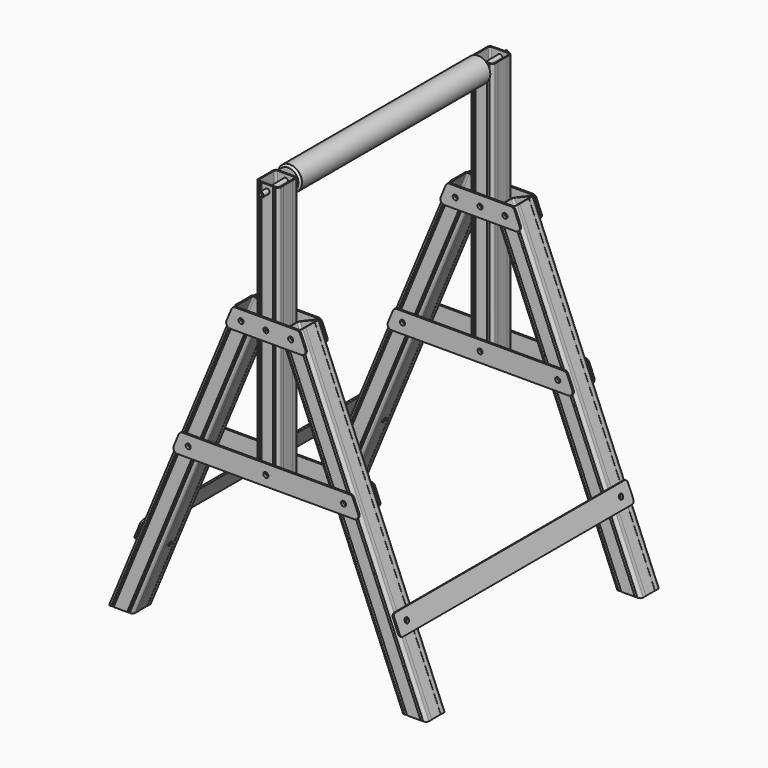
from build123d import *

# Parameters (mm, degrees)
F0_R      = 6.25
F1_DEPTH  = 60
F2_R      = 7.5
F4_REACH  = 887.042655099
F5_R      = 6.25
F6_DEPTH  = 57.7
F7_W      = 55.7
F7_H      = 653.8274706661
F7_R      = 6.25
F8_DEPTH  = 60
F9_R      = 7.5
F11_DEPTH = 653.8274706661
F14_R     = 6.25
F15_DEPTH = 4
F16_R     = 10
F16_2_R   = 10
F21_R     = 5.9
F22_DEPTH = 380
F23_R     = 30
F23_R_2   = 6.25
F24_DEPTH = 295
F25_SIZE  = 2
F26_SIZE  = 5
F28_W     = 720
F28_H     = 50
F28_R     = 6.25
F29_DEPTH = 4
F30_R     = 7.5


# Not quite as in the source:
# - a feature names something its author has since deleted; it is built from what else it names


with BuildPart() as f1:
    # F0 (on Front) → F1 (new body)
    with BuildSketch(Plane.XZ):
        Polygon((-62.4540299569, 0), (0, 0), (-310.7389470805, 750.1901803992), (-364.0467961064, 728.1093463517), align=None)
        with Locations((-201.5402531038, 411.1725293339)):
            Circle(F0_R, mode=Mode.SUBTRACT)
        with Locations((-331.6526201079, 725.2915703878)):
            Circle(F0_R, mode=Mode.SUBTRACT)
    extrude(amount=F1_DEPTH)

    # F2
    f2_edges = [f1.edges().sort_by_distance(p)[0] for p in [
        (-155.369474, -60, 375.09509),
        (-213.250413, -60, 364.054673),
        (-155.369474, 0, 375.09509),
        (-213.250413, 0, 364.054673),
    ]]
    fillet(f2_edges, radius=F2_R)

    f4_end = f1.faces().sort_by_distance((-31.2270149784, -30, 0))[0]
    # F3 (on face) → F4 (cut, up to a face of the model that its end follows)
    with BuildSketch(Plane(origin=(-310.7389470805, 0, 750.1901803992), x_dir=(0.9238795325, 0, 0.3826834324), z_dir=(-0.3826834324, 0, 0.9238795325))):
        with BuildLine():
            Line((-54.8, -30), (-54.8, -52.5))
            ThreePointArc((-54.8, -52.5), (-53.4526911935, -55.7526911935), (-50.2, -57.1))
            Line((-50.2, -57.1), (-28.85, -57.1))
            Line((-28.85, -57.1), (-7.5, -57.1))
            ThreePointArc((-7.5, -57.1), (-4.2473088065, -55.7526911935), (-2.9, -52.5))
            Line((-2.9, -52.5), (-2.9, -30))
            Line((-2.9, -30), (-2.9, -7.5))
            ThreePointArc((-2.9, -7.5), (-4.2473088065, -4.2473088065), (-7.5, -2.9))
            Line((-7.5, -2.9), (-28.85, -2.9))
            Line((-28.85, -2.9), (-50.2, -2.9))
            ThreePointArc((-50.2, -2.9), (-53.4526911935, -4.2473088065), (-54.8, -7.5))
            Line((-54.8, -7.5), (-54.8, -30))
        make_face()
        Polygon((-44.2, 0), (-46.2, 0), (-45.2, -1), align=None)
        Polygon((-46.2, 0), (-48.2, 0), (-47.2, -1), align=None)
        Polygon((-48.2, 0), (-50.2, 0), (-49.2, -1), align=None)
        Polygon((-57.7, -16), (-57.7, -44), (-57.4, -44), (-57.4, -30), (-57.4, -16), align=None)
        Polygon((-49.2, -59), (-50.2, -60), (-48.2, -60), align=None)
        Polygon((-47.2, -59), (-48.2, -60), (-46.2, -60), align=None)
        Polygon((-45.2, -59), (-46.2, -60), (-44.2, -60), align=None)
        Polygon((-8.5, -59), (-9.5, -60), (-7.5, -60), align=None)
        Polygon((-10.5, -59), (-11.5, -60), (-9.5, -60), align=None)
        Polygon((-12.5, -59), (-13.5, -60), (-11.5, -60), align=None)
        Polygon((-0.3, -44), (0, -44), (0, -16), (-0.3, -16), (-0.3, -30), align=None)
        Polygon((-7.5, 0), (-9.5, 0), (-8.5, -1), align=None)
        Polygon((-9.5, 0), (-11.5, 0), (-10.5, -1), align=None)
        Polygon((-11.5, 0), (-13.5, 0), (-12.5, -1), align=None)
    f4_long = extrude(amount=-F4_REACH, mode=Mode.PRIVATE)
    add(split(f4_long, bisect_by=f4_end, keep=Keep.BOTTOM, mode=Mode.PRIVATE), mode=Mode.SUBTRACT)

    # F5 (on face) → F6 (cut, through all)
    with BuildSketch(Plane(origin=(0, 0, 0), x_dir=(0, 1, 0), z_dir=(0.9238795325, 0, 0.3826834324))):
        with Locations((-30, 200)):
            Circle(F5_R)
    extrude(amount=-F6_DEPTH, mode=Mode.SUBTRACT)


with BuildPart() as f8:
    # F7 (on face) → F8 (new body)
    with BuildSketch(Plane.XZ.offset(60)):
        with Locations((-392.8967961064, 713.086264667)):
            Rectangle(F7_W, F7_H)
        with Locations((-392.8967961064, 411.1725293339)):
            Circle(F7_R, mode=Mode.SUBTRACT)
        with Locations((-392.8967961064, 725.2915703878)):
            Circle(F7_R, mode=Mode.SUBTRACT)
        with Locations((-392.8967961064, 1025)):
            Circle(F7_R, mode=Mode.SUBTRACT)
    extrude(amount=-F8_DEPTH)

    # F9
    f9_edges = [f8.edges().sort_by_distance(p)[0] for p in [
        (-420.746796, -60, 713.086265),
        (-365.046796, -60, 713.086265),
        (-365.046796, 0, 713.086265),
        (-420.746796, 0, 713.086265),
    ]]
    fillet(f9_edges, radius=F9_R)

    # F10 (on face) → F11 (cut, through all)
    with BuildSketch(Plane.XY.offset(1040)):
        Polygon((-412.2467961064, -59), (-413.2467961064, -60), (-411.2467961064, -60), align=None)
        Polygon((-410.2467961064, -59), (-411.2467961064, -60), (-409.2467961064, -60), align=None)
        Polygon((-408.2467961064, -59), (-409.2467961064, -60), (-407.2467961064, -60), align=None)
        Polygon((-377.5467961064, -59), (-378.5467961064, -60), (-376.5467961064, -60), align=None)
        Polygon((-375.5467961064, -59), (-376.5467961064, -60), (-374.5467961064, -60), align=None)
        Polygon((-373.5467961064, -59), (-374.5467961064, -60), (-372.5467961064, -60), align=None)
        Polygon((-420.7467961064, -16), (-420.7467961064, -44), (-420.4467961064, -44), (-420.4467961064, -30), (-420.4467961064, -16), align=None)
        Polygon((-365.3467961064, -44), (-365.0467961064, -44), (-365.0467961064, -16), (-365.3467961064, -16), (-365.3467961064, -30), align=None)
        Polygon((-376.5467961064, 0), (-378.5467961064, 0), (-377.5467961064, -1), align=None)
        Polygon((-374.5467961064, 0), (-376.5467961064, 0), (-375.5467961064, -1), align=None)
        Polygon((-372.5467961064, 0), (-374.5467961064, 0), (-373.5467961064, -1), align=None)
        Polygon((-411.2467961064, 0), (-413.2467961064, 0), (-412.2467961064, -1), align=None)
        Polygon((-409.2467961064, 0), (-411.2467961064, 0), (-410.2467961064, -1), align=None)
        Polygon((-407.2467961064, 0), (-409.2467961064, 0), (-408.2467961064, -1), align=None)
        with BuildLine():
            Line((-417.8467961064, -30), (-417.8467961064, -52.5))
            ThreePointArc((-417.8467961064, -52.5), (-416.4994872998, -55.7526911935), (-413.2467961064, -57.1))
            Line((-413.2467961064, -57.1), (-392.8967961064, -57.1))
            Line((-392.8967961064, -57.1), (-372.5467961064, -57.1))
            ThreePointArc((-372.5467961064, -57.1), (-369.2941049129, -55.7526911935), (-367.9467961064, -52.5))
            Line((-367.9467961064, -52.5), (-367.9467961064, -30))
            Line((-367.9467961064, -30), (-367.9467961064, -7.5))
            ThreePointArc((-367.9467961064, -7.5), (-369.2941049129, -4.2473088065), (-372.5467961064, -2.9))
            Line((-372.5467961064, -2.9), (-392.8967961064, -2.9))
            Line((-392.8967961064, -2.9), (-413.2467961064, -2.9))
            ThreePointArc((-413.2467961064, -2.9), (-416.4994872998, -4.2473088065), (-417.8467961064, -7.5))
            Line((-417.8467961064, -7.5), (-417.8467961064, -30))
        make_face()
    extrude(amount=-F11_DEPTH, mode=Mode.SUBTRACT)


with BuildPart() as f13_1:
    # F13: instance of F1
    add(f1.part.mirror(Plane(origin=(-392.8967961064, -30, 713.086264667), x_dir=(0, 1, 0), z_dir=(1, 0, 0))))


with BuildPart() as f15:
    # F14 (on face) → F15 (new body)
    with BuildSketch(Plane.XZ.offset(60)):
        Polygon((-180.6685771847, 436.1725293339), (-605.125015028, 436.1725293339), (-625.8356931467, 386.1725293339), (-159.957899066, 386.1725293339), align=None)
        with Locations((-584.2533391089, 411.1725293339)):
            Circle(F14_R, mode=Mode.SUBTRACT)
        with Locations((-392.8967961064, 411.1725293339)):
            Circle(F14_R, mode=Mode.SUBTRACT)
        with Locations((-201.5402531038, 411.1725293339)):
            Circle(F14_R, mode=Mode.SUBTRACT)
    extrude(amount=F15_DEPTH)

    # F16
    f16_edges = [f15.edges().sort_by_distance(p)[0] for p in [
        (-625.835693, -62, 386.172529),
        (-605.125015, -62, 436.172529),
        (-180.668577, -62, 436.172529),
        (-159.957899, -62, 386.172529),
    ]]
    fillet(f16_edges, radius=F16_R)


with BuildPart() as f15b:
    # F14 (on face) → F15, piece 2 (new body)
    with BuildSketch(Plane.XZ.offset(60)):
        Polygon((-310.7389470805, 750.1901803992), (-475.0546451323, 750.1901803992), (-495.7653232509, 700.1901803992), (-290.0282689618, 700.1901803992), align=None)
        with Locations((-454.1409721048, 725.2915703878)):
            Circle(F14_R, mode=Mode.SUBTRACT)
        with Locations((-392.8967961064, 725.1901803992)):
            Circle(F14_R, mode=Mode.SUBTRACT)
        with Locations((-331.6526201079, 725.2915703878)):
            Circle(F14_R, mode=Mode.SUBTRACT)
    extrude(amount=F15_DEPTH)

    # F16#2
    f16_2_edges = [f15b.edges().sort_by_distance(p)[0] for p in [
        (-475.054645, -62, 750.19018),
        (-495.765323, -62, 700.19018),
        (-310.738947, -62, 750.19018),
        (-290.028269, -62, 700.19018),
    ]]
    fillet(f16_2_edges, radius=F16_2_R)


with BuildPart() as f18_1:
    # F18: instance of F15
    add(f15.part.mirror(Plane(origin=(-392.8967961064, -30, 712.9824259225), x_dir=(1, 0, 0), z_dir=(0, -1, 0))))


with BuildPart() as f18_2:
    # F18: instance of F15b
    add(f15b.part.mirror(Plane(origin=(-392.8967961064, -30, 712.9824259225), x_dir=(1, 0, 0), z_dir=(0, -1, 0))))


with BuildPart() as f20_1:
    # F20: instance of F1
    add(f1.part.mirror(Plane(origin=(-392.8967961064, -360, 712.9381401651), x_dir=(1, 0, 0), z_dir=(0, -1, 0))))


with BuildPart() as f20_2:
    # F20: instance of F18_2
    add(f18_2.part.mirror(Plane(origin=(-392.8967961064, -360, 712.9381401651), x_dir=(1, 0, 0), z_dir=(0, -1, 0))))


with BuildPart() as f20_3:
    # F20: instance of F8
    add(f8.part.mirror(Plane(origin=(-392.8967961064, -360, 712.9381401651), x_dir=(1, 0, 0), z_dir=(0, -1, 0))))


with BuildPart() as f20_4:
    # F20: instance of F13_1
    add(f13_1.part.mirror(Plane(origin=(-392.8967961064, -360, 712.9381401651), x_dir=(1, 0, 0), z_dir=(0, -1, 0))))


with BuildPart() as f20_5:
    # F20: instance of F15
    add(f15.part.mirror(Plane(origin=(-392.8967961064, -360, 712.9381401651), x_dir=(1, 0, 0), z_dir=(0, -1, 0))))


with BuildPart() as f20_6:
    # F20: instance of F15b
    add(f15b.part.mirror(Plane(origin=(-392.8967961064, -360, 712.9381401651), x_dir=(1, 0, 0), z_dir=(0, -1, 0))))


with BuildPart() as f20_7:
    # F20: instance of F18_1
    add(f18_1.part.mirror(Plane(origin=(-392.8967961064, -360, 712.9381401651), x_dir=(1, 0, 0), z_dir=(0, -1, 0))))


with BuildPart() as f22:
    # F21 (on offset) → F22 (new body, symmetric)
    with BuildSketch(Plane.XZ.offset(360)):
        with Locations((-392.8967961064, 1025)):
            Circle(F21_R)
    extrude(amount=F22_DEPTH, both=True)

    # F25
    f25_edges = [f22.edges().sort_by_distance(p)[0] for p in [
        (-398.796796, 20, 1025),
        (-398.796796, -740, 1025),
    ]]
    chamfer(f25_edges, length=F25_SIZE)


with BuildPart() as f24:
    # F23 (on offset) → F24 (new body, symmetric)
    with BuildSketch(Plane.XZ.offset(360)):
        with Locations((-392.8967961064, 1025)):
            Circle(F23_R)
        with Locations((-392.8967961064, 1025)):
            Circle(F23_R_2, mode=Mode.SUBTRACT)
    extrude(amount=F24_DEPTH, both=True)

    # F26
    f26_edges = [f24.edges().sort_by_distance(p)[0] for p in [
        (-422.896796, -655, 1025),
        (-422.896796, -65, 1025),
    ]]
    chamfer(f26_edges, length=F26_SIZE)


with BuildPart() as f29:
    # F28 (on face) → F29 (new body)
    with BuildSketch(Plane(origin=(0, 0, 0), x_dir=(0, 1, 0), z_dir=(0.9238795325, 0, 0.3826834324))):
        with Locations((-360, 200)):
            Rectangle(F28_W, F28_H)
        with Locations((-690, 200)):
            Circle(F28_R, mode=Mode.SUBTRACT)
        with Locations((-30, 200)):
            Circle(F28_R, mode=Mode.SUBTRACT)
    extrude(amount=F29_DEPTH)

    # F30
    f30_edges = [f29.edges().sort_by_distance(p)[0] for p in [
        (-84.256013, 0, 208.638262),
        (-65.121842, 0, 162.444285),
        (-84.256013, -720, 208.638262),
        (-65.121842, -720, 162.444285),
    ]]
    fillet(f30_edges, radius=F30_R)


with BuildPart() as f31_1:
    # F31: instance of F29
    add(f29.part.mirror(Plane(origin=(-392.8967961064, -30, 713.086264667), x_dir=(0, 1, 0), z_dir=(1, 0, 0))))


solid = Compound([f1.part, f8.part, f13_1.part, f15.part, f15b.part, f18_1.part, f18_2.part, f20_1.part, f20_2.part, f20_3.part, f20_4.part, f20_5.part, f20_6.part, f20_7.part, f22.part, f24.part, f29.part, f31_1.part])
